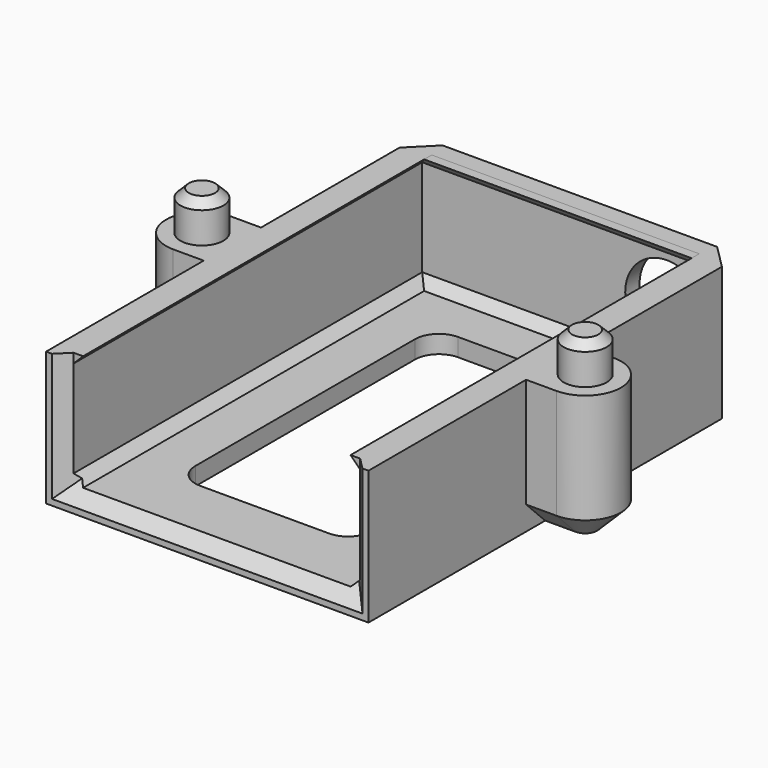
from build123d import *

# Parameters (mm, degrees)
F0_W      = 24
F0_H      = 1.5
F0_H_2    = 37.5
F0_W_2    = 14.8
F0_H_3    = 27
F1_DEPTH  = 1.5
F0_R      = 1.8
F2_DEPTH  = 11.2
F3_DEPTH  = 14.5
F4_SIZE   = 0.7
F5_DEPTH  = 11.2
F6_DEPTH  = 1.5
F7_SIZE   = 1
F8_R      = 2
F10_SIZE  = 2
F12_W     = 36.5
F12_H     = 0.8
F13_DEPTH = 0.8
F11_W     = 36.5
F11_H     = 0.8
F14_DEPTH = 0.8
F15_SIZE  = 0.79999
F9_R      = 3.5
F16_DEPTH = 1.5
F18_DEPTH = 0.8
F19_SIZE  = 0.79999


# Not quite as in the source:
# - a fillet or chamfer is up to 0.001 mm smaller than in the source, because OpenCascade refuses the exact size
# - ends of sketch curves that miss each other by under 0.0002 mm in the source are joined


with BuildPart() as f1:
    # F0 (on Top) → F1 (new body)
    with BuildSketch(Plane.XY):
        with Locations((0, 18.75)):
            Rectangle(F0_W, F0_H)
        with Locations((0, -0.75)):
            Rectangle(F0_W, F0_H_2)
        Rectangle(F0_W_2, F0_H_3, mode=Mode.SUBTRACT)
    extrude(amount=F1_DEPTH)

    # F0 (on Top) → F2 (join)
    with BuildSketch(Plane.XY):
        with BuildLine():
            Line((-13.5, 3), (-16.05, 3))
            ThreePointArc((-16.05, 3), (-19.05, 0), (-16.05, -3))
            Line((-16.05, -3), (-13.5, -3))
            Line((-13.5, -3), (-13.5, 3))
        make_face()
        with Locations((-16.05, 0)):
            Circle(F0_R, mode=Mode.SUBTRACT)
        with Locations((-16.05, 0)):
            Circle(F0_R)
        Polygon((-13.5, 19.5), (-13.5, 3), (-13.5, -3), (-13.5, -19.5), (-12, -19.5), (-12, 18), (-12, 19.5), align=None)
        with BuildLine():
            Line((16.05, 3), (13.5, 3))
            Line((13.5, 3), (13.5, -3))
            Line((13.5, -3), (16.05, -3))
            ThreePointArc((16.05, -3), (19.05, 0), (16.05, 3))
        make_face()
        with Locations((16.05, 0)):
            Circle(F0_R, mode=Mode.SUBTRACT)
        with Locations((16.05, 0)):
            Circle(F0_R)
        Polygon((13.5, 19.5), (12, 19.5), (12, 18), (12, -19.5), (13.5, -19.5), (13.5, -3), (13.5, 3), align=None)
    extrude(amount=F2_DEPTH)

    # F0 (on Top) → F3 (join)
    with BuildSketch(Plane.XY):
        with Locations((-16.05, 0)):
            Circle(F0_R)
        with Locations((16.05, 0)):
            Circle(F0_R)
    extrude(amount=F3_DEPTH)

    # F4
    f4_edges = [f1.edges().sort_by_distance(p)[0] for p in [
        (14.25, 0, 14.5),
        (-17.85, 0, 14.5),
    ]]
    chamfer(f4_edges, length=F4_SIZE)

    # F0 (on Top) → F5 (join, through all)
    with BuildSketch(Plane.XY):
        with Locations((0, 18.75)):
            Rectangle(F0_W, F0_H)
    extrude(amount=F5_DEPTH)

    # F0 (on Top) → F6 (join)
    with BuildSketch(Plane.XY):
        with Locations((0, -0.75)):
            Rectangle(F0_W, F0_H_2)
        Rectangle(F0_W_2, F0_H_3, mode=Mode.SUBTRACT)
    extrude(amount=F6_DEPTH)

    # F7
    f7_edges = [f1.edges().sort_by_distance(p)[0] for p in [
        (12, -19.5, 6.35),
        (0, -19.5, 1.5),
        (-12, -19.5, 6.35),
    ]]
    chamfer(f7_edges, length=F7_SIZE)

    # F8
    f8_edges = [f1.edges().sort_by_distance(p)[0] for p in [
        (7.4, 13.5, 0.75),
        (-7.4, 13.5, 0.75),
        (7.4, -13.5, 0.75),
        (-7.4, -13.5, 0.75),
    ]]
    fillet(f8_edges, radius=F8_R)

    # F10
    f10_edges = [f1.edges().sort_by_distance(p)[0] for p in [
        (13.5, 19.5, 5.6),
        (-13.5, 19.5, 5.6),
        (19.05, 0, 0),
        (-19.05, 0, 0),
    ]]
    chamfer(f10_edges, length=F10_SIZE)

    # F12 (on face) → F13 (join)
    with BuildSketch(Plane(origin=(12, 0, 0), x_dir=(0, -1, 0), z_dir=(-1, 0, 0))):
        with Locations((0.25, 10.8)):
            Rectangle(F12_W, F12_H)
    extrude(amount=F13_DEPTH)

    # F11 (on face) → F14 (join)
    with BuildSketch(Plane.YZ.offset(-12)):
        with Locations((-0.25, 10.8)):
            Rectangle(F11_W, F11_H)
    extrude(amount=F14_DEPTH)

    # F15 (size 0.8 in the source; OpenCascade refuses exactly that, so slightly less here)
    f15_edges = [f1.edges().sort_by_distance(p)[0] for p in [
        (-11.2, -0.25, 10.4),
        (11.2, -0.25, 10.4),
        (-12, -0.25, 1.5),
        (12, -0.25, 1.5),
        (0, 18, 1.5),
    ]]
    chamfer(f15_edges, length=F15_SIZE)

    # F9 (on face) → F16 (cut)
    with BuildSketch(Plane(origin=(0, 19.5, 0), x_dir=(-1, 0, 0), z_dir=(0, 1, 0))):
        with Locations((-8.5, 6.35)):
            Circle(F9_R)
    extrude(amount=-F16_DEPTH, mode=Mode.SUBTRACT)

    # F17 (on face) → F18 (join)
    with BuildSketch(Plane.XZ.offset(-18)):
        Polygon((-12, 10.4), (12, 10.4), (11.2, 11.19999), (-11.2, 11.2), align=None)
    extrude(amount=F18_DEPTH)

    # F19 (size 0.8 in the source; OpenCascade refuses exactly that, so slightly less here)
    f19_edges = [f1.edges().sort_by_distance(p)[0] for p in [
        (0, 17.2, 10.4),
    ]]
    chamfer(f19_edges, length=F19_SIZE)


with BuildPart() as f20_1:
    # F20: copy of F1
    add(f1.part)


solid = Compound([f1.part, f20_1.part])
